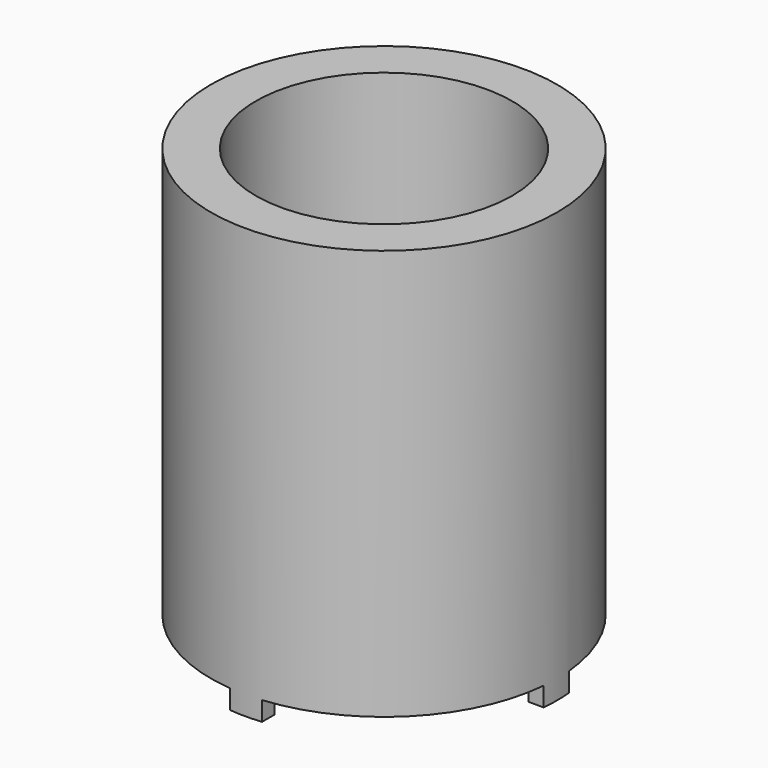
from build123d import *

# Parameters (mm, degrees)
F0_R            = 85.725
F0_R_2          = 63.5
F1_DEPTH        = 203.2
F3_DEPTH        = 9.525
F3_COPIES_COUNT = 4


# Not quite as in the source:
# - after a boolean that leaves OpenCascade's solid faulty, fix() repairs it
# - a pattern or mirror of a feature is missing from the dataset's text; its kind, count and spacing are read off the source's solid


with BuildPart() as f1:
    # F0 (on Top) → F1 (new body)
    with BuildSketch(Plane.XY):
        Circle(F0_R)
        Circle(F0_R_2, mode=Mode.SUBTRACT)
    extrude(amount=F1_DEPTH)

    # F2 (on face) → F3 (join)
    with BuildSketch(Plane(origin=(0, 0, 0), x_dir=(1, 0, 0), z_dir=(0, 0, -1))):
        with BuildLine():
            Line((-7.874, 85.3626132976), (-7.874, 77.7426132976))
            Line((-7.874, 77.7426132976), (7.874, 77.7426132976))
            Line((7.874, 77.7426132976), (7.874, 85.3626132976))
            ThreePointArc((7.874, 85.3626132976), (0, 85.725), (-7.874, 85.3626132976))
        make_face()
    f3 = extrude(amount=F3_DEPTH)

    # F3_copies: F3 ×4 about axis
    f3_copies_axis = Axis((0, 0, 0), (0, 0, 1))
    for i in range(1, F3_COPIES_COUNT):
        add(f3.rotate(f3_copies_axis, i * 360 / F3_COPIES_COUNT))

    add(f1.part.fix(), mode=Mode.REPLACE)


solid = f1.part
